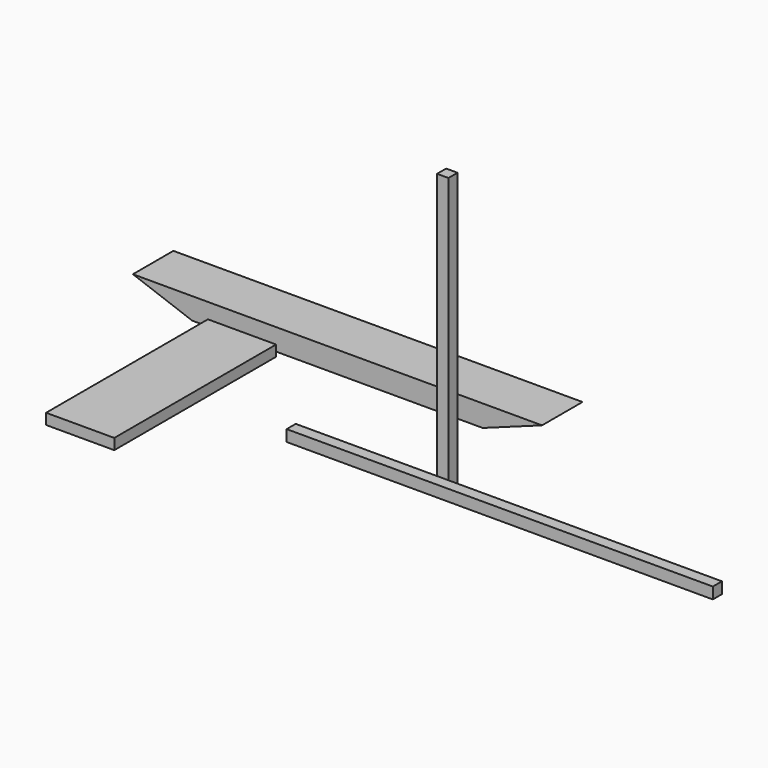
from build123d import *

# Parameters (mm, degrees)
F0_W       = 720
F0_H       = 89
F1_DEPTH   = 19
F2_W       = 120
F2_H       = 356
F3_DEPTH   = 9.5
F4_SIZE2   = 104.404132
F4_SIZE    = 37.99999
F4_2_SIZE2 = 104.404132
F4_2_SIZE  = 37.99999
F5_W       = 20
F5_H       = 500
F6_DEPTH   = 20
F7_W       = 750
F7_H       = 20
F8_DEPTH   = 20


# Not quite as in the source:
# - a fillet or chamfer is up to 0.001 mm smaller than in the source, because OpenCascade refuses the exact size


with BuildPart() as f1:
    # F0 (on Top) → F1 (new body, symmetric)
    with BuildSketch(Plane.XY):
        with Locations((-16.3644044673, 44.5)):
            Rectangle(F0_W, F0_H)
    extrude(amount=F1_DEPTH, both=True)

    # F4 (size 38 and 104.4041419393 in the source; OpenCascade refuses exactly that, so slightly less here)
    f4_edges = [f1.edges().sort_by_distance(p)[0] for p in [
        (-376.364404, 44.5, -19),
    ]]
    f4_side = f1.faces().sort_by_distance((-376.364404, 44.5, 0))[0]
    chamfer(f4_edges, length=F4_SIZE, length2=F4_SIZE2, reference=f4_side)

    # F4#2 (size 38 and 104.4041419393 in the source; OpenCascade refuses exactly that, so slightly less here)
    f4_2_edges = [f1.edges().sort_by_distance(p)[0] for p in [
        (343.635596, 44.5, -19),
    ]]
    f4_2_side = f1.faces().sort_by_distance((343.635596, 44.5, 0))[0]
    chamfer(f4_2_edges, length=F4_2_SIZE, length2=F4_2_SIZE2, reference=f4_2_side)


with BuildPart() as f3:
    # F2 (on Top) → F3 (new body, symmetric)
    with BuildSketch(Plane.XY):
        with Locations((-163.3983030915, -204.1987112857)):
            Rectangle(F2_W, F2_H)
    extrude(amount=F3_DEPTH, both=True)


with BuildPart() as f6:
    # F5 (on Front) → F6 (new body)
    with BuildSketch(Plane.XZ):
        with Locations((184.8932749033, 111.9590550661)):
            Rectangle(F5_W, F5_H)
    extrude(amount=F6_DEPTH)


with BuildPart() as f8:
    # F7 (on Top) → F8 (new body)
    with BuildSketch(Plane.XY):
        with Locations((452.7677640198, -219.4832157493)):
            Rectangle(F7_W, F7_H)
    extrude(amount=F8_DEPTH)


solid = Compound([f1.part, f3.part, f6.part, f8.part])
